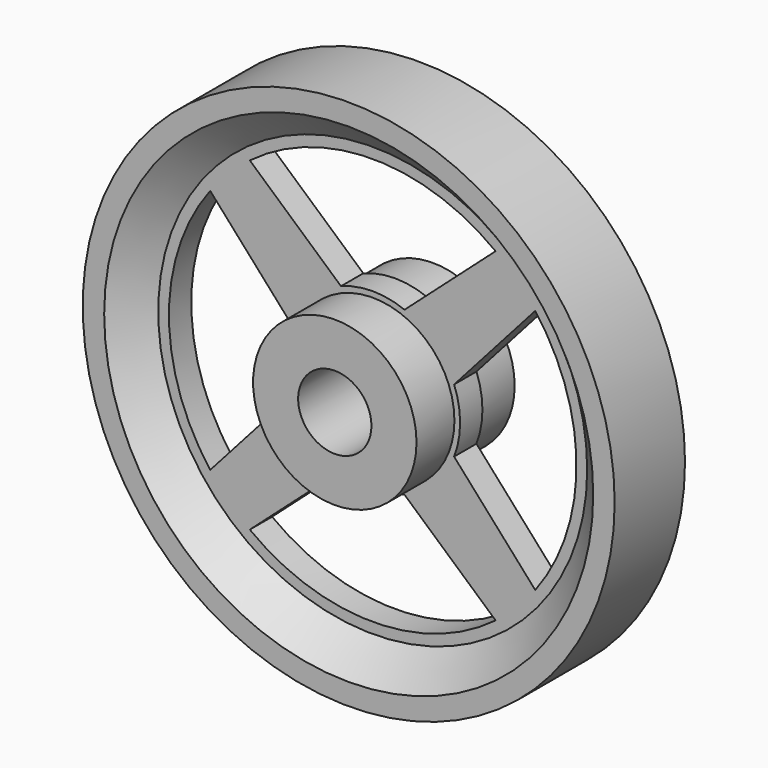
from build123d import *

# Parameters (mm, degrees)
F0_R     = 38.095
F0_R_2   = 17.08
F1_DEPTH = 28.6
F0_R_3   = 100
F2_DEPTH = 6.5
F0_R_4   = 114
F3_DEPTH = 20.5
F4_SIZE  = 13.99999
F0_R_5   = 124
F5_DEPTH = 20.5


# Not quite as in the source:
# - a fillet or chamfer is up to 0.001 mm smaller than in the source, because OpenCascade refuses the exact size


with BuildPart() as f1:
    # F0 (on Front) → F1 (new body, symmetric)
    with BuildSketch(Plane.XZ):
        Circle(F0_R)
        Circle(F0_R_2, mode=Mode.SUBTRACT)
    extrude(amount=F1_DEPTH, both=True)

    # F0 (on Front) → F2 (join, symmetric)
    with BuildSketch(Plane.XZ):
        Circle(F0_R_3)
        with BuildLine():
            Line((-57.3000000001, -75.7740720829), (-14.84, -37.9464020034))
            ThreePointArc((-14.84, -37.9464020034), (-0.0346057341, -40.7449853042), (14.775520982, -37.9715552053))
            Line((14.775520982, -37.9715552053), (14.7748944579, -37.9464020034))
            Line((14.7748944579, -37.9464020034), (14.7947522966, -37.9640662928))
            Line((14.7947522966, -37.9640662928), (57.2999999977, -75.7740720847))
            ThreePointArc((57.2999999977, -75.7740720847), (-1.5e-09, -95.0000000002), (-57.3000000001, -75.7740720829))
        make_face(mode=Mode.SUBTRACT)
        with BuildLine():
            Line((75.7740720829, -57.3), (37.9464020034, -14.84))
            ThreePointArc((37.9464020034, -14.84), (40.7449927617, -0.0242867339), (37.9640662928, 14.7947522966))
            Line((37.9640662928, 14.7947522966), (75.7740720847, 57.2999999977))
            ThreePointArc((75.7740720847, 57.2999999977), (95.0000000002, -1.5e-09), (75.7740720829, -57.3))
        make_face(mode=Mode.SUBTRACT)
        with BuildLine():
            ThreePointArc((-75.7740720847, -57.2999999977), (-95.0000000002, 1.5e-09), (-75.7740720829, 57.3000000001))
            Line((-75.7740720829, 57.3), (-37.9464020034, 14.84))
            ThreePointArc((-37.9464020034, 14.84), (-40.7449927617, 0.0242867339), (-37.9640662928, -14.7947522966))
            Line((-37.9640662928, -14.7947522966), (-75.7740720847, -57.2999999977))
        make_face(mode=Mode.SUBTRACT)
        Circle(F0_R, mode=Mode.SUBTRACT)
        with BuildLine():
            Line((57.3, 75.7740720829), (14.84, 37.9464020034))
            ThreePointArc((14.84, 37.9464020034), (0.0242867339, 40.7449927617), (-14.7947522966, 37.9640662928))
            Line((-14.7947522966, 37.9640662928), (-57.2999999977, 75.7740720847))
            ThreePointArc((-57.2999999977, 75.7740720847), (1.5e-09, 95.0000000002), (57.3, 75.7740720829))
        make_face(mode=Mode.SUBTRACT)
    extrude(amount=F2_DEPTH, both=True)

    # F0 (on Front) → F3 (join, symmetric)
    with BuildSketch(Plane.XZ):
        Circle(F0_R_4)
        Circle(F0_R_3, mode=Mode.SUBTRACT)
    extrude(amount=F3_DEPTH, both=True)

    # F4 (size 14 in the source; OpenCascade refuses exactly that, so slightly less here)
    f4_edges = [f1.edges().sort_by_distance(p)[0] for p in [
        (-100, -20.5, 0),
        (-100, 20.5, 0),
    ]]
    chamfer(f4_edges, length=F4_SIZE)

    # F0 (on Front) → F5 (join, symmetric)
    with BuildSketch(Plane.XZ):
        Circle(F0_R_5)
        Circle(F0_R_4, mode=Mode.SUBTRACT)
    extrude(amount=F5_DEPTH, both=True)


solid = f1.part
